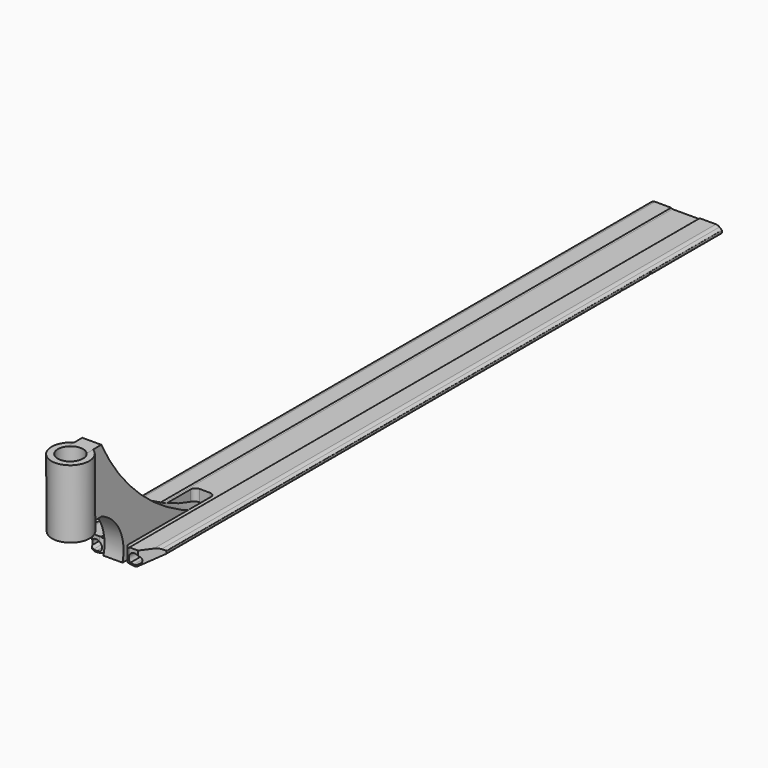
from build123d import *

# Parameters (mm, degrees)
F1_DEPTH       = 931
F1_DEPTH_BACK  = 242
F2_W           = 38
F2_H           = 13
F3_DEPTH       = 250
F4_T1_DEPTH    = 1173
F5_R           = 9
F6_R           = 1
F8_DEPTH       = 1173.001
F10_DEPTH      = 22.3229098862
F12_DEPTH      = 26.90495442
F13_T4_DEPTH   = 40.1407788292
F13_S5_R       = 200
F13_T6_DEPTH   = 22
F13_T10_DEPTH  = 39.9941485469
F13_S11_R      = 200
F13_T12_DEPTH  = 22
F13_T13_DEPTH  = 59.4544873282
F13_T15_DEPTH  = 59.3078570459
F14_R          = 3.131898342
F15_DEPTH      = 89
F15_DEPTH_BACK = 62
F17_DEPTH      = 15
F19_DEPTH      = 108
F21_D          = 40


# Not quite as in the source:
# - a fillet or chamfer that OpenCascade refuses, or shapes differently, is made with other operations: its cross-section is extruded or revolved along the edge and cut away or added


with BuildPart() as f1:
    # F0 (on Front) → F1 (new body, two sides)
    with BuildSketch(Plane.XZ) as f1_sk:
        with BuildLine():
            Line((22.5, 25.60395442), (0, 25.60395442))
            Line((0, 25.60395442), (-22.5, 25.60395442))
            Line((-22.5, 25.60395442), (-22.5, 26.90395442))
            Line((-22.5, 26.90395442), (-51.1562512645, 26.90395442))
            Line((-51.1562512645, 26.90395442), (-57.5, 21.5809171957))
            Line((-57.5, 21.5809171957), (-57.5, 17.5809171957))
            Line((-57.5, 17.5809171957), (-32.0787547716, 2.90395442))
            ThreePointArc((-32.0787547716, 2.90395442), (0, 5.4933328914), (32.0787547716, 2.90395442))
            Line((32.0787547716, 2.90395442), (57.5, 17.5809171957))
            Line((57.5, 17.5809171957), (57.5, 21.5809171957))
            Line((57.5, 21.5809171957), (51.1562512645, 26.90395442))
            Line((51.1562512645, 26.90395442), (22.5, 26.90395442))
            Line((22.5, 26.90395442), (22.5, 25.60395442))
        make_face()
    extrude(amount=-F1_DEPTH)
    extrude(f1_sk.sketch, amount=F1_DEPTH_BACK)

    # F2 (on face) → F3 (cut, symmetric)
    with BuildSketch(Plane(origin=(0, 931, 0), x_dir=(-1, 0, 0), z_dir=(0, 1, 0))):
        with Locations((0, 17.10395442)):
            Rectangle(F2_W, F2_H)
    extrude(amount=F3_DEPTH, both=True, mode=Mode.SUBTRACT)

    # F4: fillet of radius 2 on 2 edges, made by hand

    # F4_s2 → F4_t1 (join)
    with BuildSketch(Plane.XZ.offset(-931)):
        with BuildLine():
            ThreePointArc((-22.5, 26.90395442), (-21.7666760256, 25.9607867475), (-20.6265006005, 25.60395442))
            Line((-20.6265006005, 25.60395442), (-22.5, 25.60395442))
            Line((-22.5, 25.60395442), (-22.5, 26.90395442))
        make_face()
        with BuildLine():
            ThreePointArc((22.5, 26.90395442), (21.7666760256, 25.9607867475), (20.6265006005, 25.60395442))
            Line((20.6265006005, 25.60395442), (22.5, 25.60395442))
            Line((22.5, 25.60395442), (22.5, 26.90395442))
        make_face()
    extrude(amount=F4_T1_DEPTH)

    # F5
    f5_edges = [f1.edges().sort_by_distance(p)[0] for p in [
        (-51.156251, 344.5, 26.903954),
        (51.156251, 344.5, 26.903954),
        (-32.078755, 344.5, 2.903954),
        (32.078755, 344.5, 2.903954),
    ]]
    fillet(f5_edges, radius=F5_R)

    # F6
    f6_edges = [f1.edges().sort_by_distance(p)[0] for p in [
        (-57.5, 344.5, 21.580917),
        (-57.5, 344.5, 17.580917),
        (57.5, 344.5, 21.580917),
        (57.5, 344.5, 17.580917),
    ]]
    fillet(f6_edges, radius=F6_R)

    # F7 (on face) → F8 (cut, through all)
    with BuildSketch(Plane(origin=(0, 931, 0), x_dir=(-1, 0, 0), z_dir=(0, 1, 0))):
        with BuildLine():
            ThreePointArc((-23.7934508606, 6.0871306423), (-28.5708919173, 21.1100300712), (-38.7210628123, 9.0482938321))
            Line((-38.7210628123, 9.0482938321), (-33.8220833267, 6.2198667073))
            ThreePointArc((-33.8220833267, 6.2198667073), (-31.6372318721, 5.4066984114), (-29.3065111579, 5.3561068233))
            ThreePointArc((-29.3065111579, 5.3561068233), (-26.5524968797, 5.740592322), (-23.7934508606, 6.0871306423))
        make_face()
        with BuildLine():
            ThreePointArc((38.7210628123, 9.0482938321), (28.5708919173, 21.1100300712), (23.7934508606, 6.0871306423))
            ThreePointArc((23.7934508606, 6.0871306423), (26.5524968797, 5.740592322), (29.3065111579, 5.3561068233))
            ThreePointArc((29.3065111579, 5.3561068233), (31.6372318721, 5.4066984114), (33.8220833267, 6.2198667073))
            Line((33.8220833267, 6.2198667073), (38.7210628123, 9.0482938321))
        make_face()
    extrude(amount=-F8_DEPTH, mode=Mode.SUBTRACT)

    # F9 (on face) → F10 (cut, through all)
    with BuildSketch(Plane.XY.offset(25.60395442)):
        with BuildLine():
            ThreePointArc((-57.5, -292), (0.0986348044, -234.5000845985), (57.4996616061, -292.1972693185))
            Line((57.4996616061, -292.1972693185), (57.7741248818, -212.1972693185))
            Line((57.7741248818, -212.1972693185), (-57.5, -212.1972693185))
            Line((-57.5, -212.1972693185), (-57.5, -292))
        make_face()
    extrude(amount=-F10_DEPTH, mode=Mode.SUBTRACT)

    # F11 (on Top) → F12 (cut, through all)
    with BuildSketch(Plane.XY):
        Polygon((-68.1919046547, -149.9935638406), (-68.1919046547, -249.9935638406), (67.8080953453, -249.9935638406), (67.8080953453, -149.9935638406), (36.0676917215, -193.6804815369), (15.0865076999, -193.6804815369), (15.0865076999, -16), (-16.9134923001, -16), (-16.9134923001, -193.6804815369), (-36.4515010309, -193.6804815369), align=None)
    extrude(amount=F12_DEPTH, mode=Mode.SUBTRACT)

    # F13: fillet of radius 7.7254833996 on 4 edges, made by hand


with BuildPart() as f13_tool2:
    # F13_s3 → F13_t4 (new body)
    with BuildSketch(Plane.XY.offset(-14.5368244092)):
        with BuildLine():
            ThreePointArc((-16.9134923001, -23.7254833996), (-14.6507506003, -18.2627416998), (-9.1880089005, -16))
            Line((-9.1880089005, -16), (-16.9134923001, -16))
            Line((-16.9134923001, -16), (-16.9134923001, -23.7254833996))
        make_face()
    extrude(amount=F13_T4_DEPTH)

    # F13_s5 → F13_t6 (cut, symmetric)
    with BuildSketch(Plane.XZ.offset(19.9)):
        with Locations((0, -194.5066671086)):
            Circle(F13_S5_R)
    extrude(amount=F13_T6_DEPTH, both=True, mode=Mode.SUBTRACT)


with BuildPart() as f1_1:
    add(f1.part)

    # F13_t1: union F13_tool2
    add(f13_tool2.part)


with BuildPart() as f13_tool8:
    # F13_s9 → F13_t10 (new body)
    with BuildSketch(Plane.XY.offset(-14.3901941269)):
        with BuildLine():
            ThreePointArc((7.3610243003, -16), (12.8237660001, -18.2627416998), (15.0865076999, -23.7254833996))
            Line((15.0865076999, -23.7254833996), (15.0865076999, -16))
            Line((15.0865076999, -16), (7.3610243003, -16))
        make_face()
    extrude(amount=F13_T10_DEPTH)

    # F13_s11 → F13_t12 (cut, symmetric)
    with BuildSketch(Plane.XZ.offset(19.9)):
        with Locations((0, -194.5066671086)):
            Circle(F13_S11_R)
    extrude(amount=F13_T12_DEPTH, both=True, mode=Mode.SUBTRACT)


with BuildPart() as f1_2:
    add(f1_1.part)

    # F13_t7: union F13_tool8
    add(f13_tool8.part)

    # F13_s14 → F13_t13 (cut)
    with BuildSketch(Plane.XY.offset(-14.5368244092)):
        with BuildLine():
            ThreePointArc((-24.6389756997, -193.6804815369), (-19.1762339999, -191.4177398371), (-16.9134923001, -185.9549981373))
            Line((-16.9134923001, -185.9549981373), (-16.9134923001, -193.6804815369))
            Line((-16.9134923001, -193.6804815369), (-24.6389756997, -193.6804815369))
        make_face()
    extrude(amount=F13_T13_DEPTH, mode=Mode.SUBTRACT)

    # F13_s16 → F13_t15 (cut)
    with BuildSketch(Plane.XY.offset(-14.3901941269)):
        with BuildLine():
            ThreePointArc((15.0865076999, -185.9549981373), (17.3492493997, -191.4177398371), (22.8119910995, -193.6804815369))
            Line((22.8119910995, -193.6804815369), (15.0865076999, -193.6804815369))
            Line((15.0865076999, -193.6804815369), (15.0865076999, -185.9549981373))
        make_face()
    extrude(amount=F13_T15_DEPTH, mode=Mode.SUBTRACT)

    # F14 (on face) → F15 (cut, two sides)
    with BuildSketch(Plane.YZ.offset(-19)) as f15_sk:
        with Locations((790.3922146022, 16.661236415)):
            Circle(F14_R)
        with Locations((734.131898342, 16.0354316436)):
            Circle(F14_R)
    extrude(amount=F15_DEPTH, mode=Mode.SUBTRACT)
    extrude(f15_sk.sketch, amount=-F15_DEPTH_BACK, mode=Mode.SUBTRACT)

    # F16 (on Right) → F17 (join, symmetric)
    with BuildSketch(Plane.YZ):
        with BuildLine():
            Line((-198.0922913931, 5), (-8.0922913931, 5))
            ThreePointArc((-8.0922913931, 5), (-143.995655135, 69.8938040775), (-240.0484130204, 185.8886220074))
            Line((-240.0484130204, 185.8886220074), (-286.0456626008, 185.3856000985))
            Line((-286.0456626008, 185.3856000985), (-284.9521367117, 85.3915792716))
            Line((-284.9521367117, 85.3915792716), (-238.9548871314, 85.8946011805))
            ThreePointArc((-238.9548871314, 85.8946011805), (-203.6649933497, 52.9528793205), (-198.0922913931, 5))
        make_face()
    extrude(amount=F17_DEPTH, both=True)

    # F18 (on face) → F19 (join)
    with BuildSketch(Plane(origin=(0, -2.0613236275, 188.4912280569), x_dir=(1, 0, 0), z_dir=(0, -0.0109352589, 0.9999402083))):
        with BuildLine():
            ThreePointArc((-15, -254.0765678363), (-15, -306.0380920634), (30, -280.0573299498))
            ThreePointArc((30, -280.0573299498), (25.9807621135, -265.0573299498), (15, -254.0765678363))
            Line((15, -254.0765678363), (15, -284.0013199038))
            Line((15, -284.0013199038), (-15, -284.0013199038))
            Line((-15, -284.0013199038), (-15, -254.0765678363))
        make_face()
        with BuildLine():
            Line((15, -284.0013199038), (15, -254.0765678363))
            ThreePointArc((15, -254.0765678363), (0, -250.0573299498), (-15, -254.0765678363))
            Line((-15, -254.0765678363), (-15, -284.0013199038))
            Line((-15, -284.0013199038), (15, -284.0013199038))
        make_face()
    extrude(amount=-F19_DEPTH)

    # F21 (through all)
    with Locations(Plane(origin=(0, -2.0613236275, 188.4912280569), x_dir=(1, 0, 0), z_dir=(0, -0.0109352589, 0.9999402083))):
        with Locations((0, -280.0573299498)):
            Hole(F21_D / 2)


solid = f1_2.part
